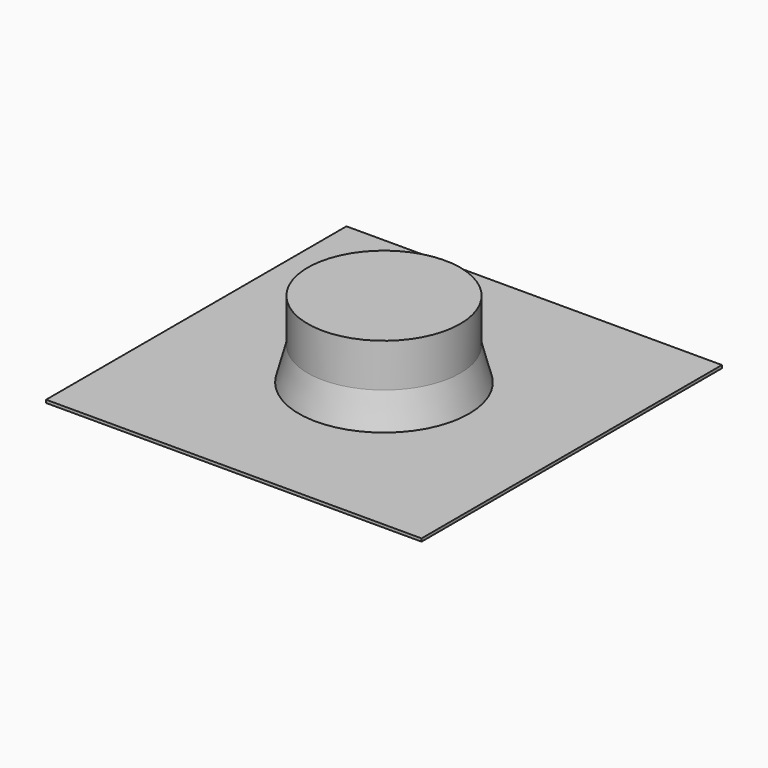
from build123d import *

# Parameters (mm, degrees)
F2_R     = 46.0375
F3_DEPTH = 19.05
F3_TAPER = 15
F0_R     = 41.275
F4_DEPTH = 25.4
F5_R     = 46.0375
F6_DEPTH = 1.5875


with BuildPart() as f3:
    # F2 (on offset) → F3 (new body)
    with BuildSketch(Plane.XY.offset(-41.275)):
        Circle(F2_R)
    extrude(amount=F3_DEPTH, taper=F3_TAPER)

    # F0 (on Top) → F4 (join)
    with BuildSketch(Plane.XY):
        Circle(F0_R)
    extrude(amount=-F4_DEPTH)

    # F5 (on face) → F6 (join)
    with BuildSketch(Plane(origin=(0, 0, -41.275), x_dir=(1, 0, 0), z_dir=(0, 0, -1))):
        Polygon((101.6, -101.6), (101.6, 0), (101.6, 101.6), (-101.6, 101.6), (-101.6, -101.6), align=None)
        Circle(F5_R, mode=Mode.SUBTRACT)
        Circle(F5_R)
    extrude(amount=F6_DEPTH)


solid = f3.part
